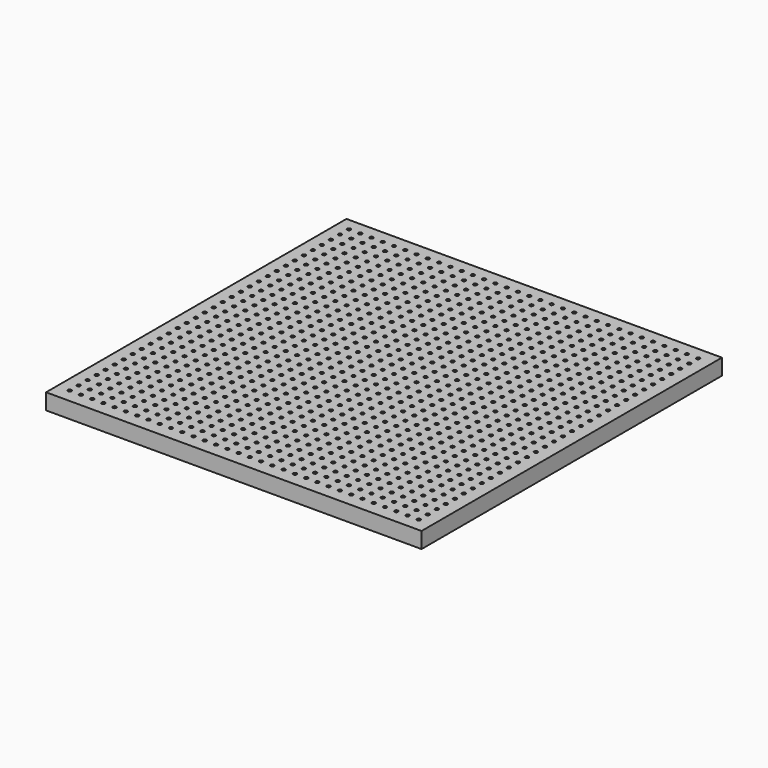
from build123d import *

# Parameters (mm, degrees)
F0_W     = 400
F0_H     = 400
F1_DEPTH = 1.5
F3_W     = 400
F3_H     = 400
F3_W_2   = 397
F3_H_2   = 397
F4_DEPTH = 15.5
F5_DEPTH = 10.5
F6_DEPTH = 10.5
F2_R     = 1.875
F7_DEPTH = 17.001


with BuildPart() as f1:
    # F0 (on Top) → F1 (new body)
    with BuildSketch(Plane.XY):
        Rectangle(F0_W, F0_H)
    extrude(amount=F1_DEPTH)

    # F3 (on face) → F4 (join)
    with BuildSketch(Plane(origin=(0, 0, 0), x_dir=(1, 0, 0), z_dir=(0, 0, -1))):
        Rectangle(F3_W, F3_H)
        Rectangle(F3_W_2, F3_H_2, mode=Mode.SUBTRACT)
    extrude(amount=F4_DEPTH)

    # F5 (add): a face of the model
    f5_faces = [f1.faces().sort_by_distance(p)[0] for p in [
        (0, -198.5, -7.75),
    ]]
    extrude(f5_faces, amount=F5_DEPTH)

    # F6 (add): a face of the model
    f6_faces = [f1.faces().sort_by_distance(p)[0] for p in [
        (0, 198.5, -7.75),
    ]]
    extrude(f6_faces, amount=F6_DEPTH)

    # F2 (on face) → F7 (cut, through all)
    with BuildSketch(Plane.XY.offset(1.5)):
        with Locations((-186.625, 186.625)):
            Circle(F2_R)
        with Locations((-186.625, 174.625)):
            Circle(F2_R)
        with Locations((-186.625, 162.625)):
            Circle(F2_R)
        with Locations((-186.625, 150.625)):
            Circle(F2_R)
        with Locations((-186.625, 138.625)):
            Circle(F2_R)
        with Locations((-186.625, 126.625)):
            Circle(F2_R)
        with Locations((-186.625, 114.625)):
            Circle(F2_R)
        with Locations((-186.625, 102.625)):
            Circle(F2_R)
        with Locations((-186.625, 90.625)):
            Circle(F2_R)
        with Locations((-186.625, 78.625)):
            Circle(F2_R)
        with Locations((-186.625, 66.625)):
            Circle(F2_R)
        with Locations((-186.625, 54.625)):
            Circle(F2_R)
        with Locations((-186.625, 42.625)):
            Circle(F2_R)
        with Locations((-186.625, 30.625)):
            Circle(F2_R)
        with Locations((-186.625, 18.625)):
            Circle(F2_R)
        with Locations((-186.625, 6.625)):
            Circle(F2_R)
        with Locations((-186.625, -5.375)):
            Circle(F2_R)
        with Locations((-186.625, -17.375)):
            Circle(F2_R)
        with Locations((-186.625, -29.375)):
            Circle(F2_R)
        with Locations((-186.625, -41.375)):
            Circle(F2_R)
        with Locations((-186.625, -53.375)):
            Circle(F2_R)
        with Locations((-186.625, -65.375)):
            Circle(F2_R)
        with Locations((-186.625, -77.375)):
            Circle(F2_R)
        with Locations((-186.625, -89.375)):
            Circle(F2_R)
        with Locations((-186.625, -101.375)):
            Circle(F2_R)
        with Locations((-186.625, -113.375)):
            Circle(F2_R)
        with Locations((-186.625, -125.375)):
            Circle(F2_R)
        with Locations((-186.625, -137.375)):
            Circle(F2_R)
        with Locations((-186.625, -149.375)):
            Circle(F2_R)
        with Locations((-186.625, -161.375)):
            Circle(F2_R)
        with Locations((-186.625, -173.375)):
            Circle(F2_R)
        with Locations((-186.625, -185.375)):
            Circle(F2_R)
        with Locations((-174.625, 186.625)):
            Circle(F2_R)
        with Locations((-174.625, 174.625)):
            Circle(F2_R)
        with Locations((-174.625, 162.625)):
            Circle(F2_R)
        with Locations((-174.625, 150.625)):
            Circle(F2_R)
        with Locations((-174.625, 138.625)):
            Circle(F2_R)
        with Locations((-174.625, 126.625)):
            Circle(F2_R)
        with Locations((-174.625, 114.625)):
            Circle(F2_R)
        with Locations((-174.625, 102.625)):
            Circle(F2_R)
        with Locations((-174.625, 90.625)):
            Circle(F2_R)
        with Locations((-174.625, 78.625)):
            Circle(F2_R)
        with Locations((-174.625, 66.625)):
            Circle(F2_R)
        with Locations((-174.625, 54.625)):
            Circle(F2_R)
        with Locations((-174.625, 42.625)):
            Circle(F2_R)
        with Locations((-174.625, 30.625)):
            Circle(F2_R)
        with Locations((-174.625, 18.625)):
            Circle(F2_R)
        with Locations((-174.625, 6.625)):
            Circle(F2_R)
        with Locations((-174.625, -5.375)):
            Circle(F2_R)
        with Locations((-174.625, -17.375)):
            Circle(F2_R)
        with Locations((-174.625, -29.375)):
            Circle(F2_R)
        with Locations((-174.625, -41.375)):
            Circle(F2_R)
        with Locations((-174.625, -53.375)):
            Circle(F2_R)
        with Locations((-174.625, -65.375)):
            Circle(F2_R)
        with Locations((-174.625, -77.375)):
            Circle(F2_R)
        with Locations((-174.625, -89.375)):
            Circle(F2_R)
        with Locations((-174.625, -101.375)):
            Circle(F2_R)
        with Locations((-174.625, -113.375)):
            Circle(F2_R)
        with Locations((-174.625, -125.375)):
            Circle(F2_R)
        with Locations((-174.625, -137.375)):
            Circle(F2_R)
        with Locations((-174.625, -149.375)):
            Circle(F2_R)
        with Locations((-174.625, -161.375)):
            Circle(F2_R)
        with Locations((-174.625, -173.375)):
            Circle(F2_R)
        with Locations((-174.625, -185.375)):
            Circle(F2_R)
        with Locations((-162.625, 186.625)):
            Circle(F2_R)
        with Locations((-162.625, 174.625)):
            Circle(F2_R)
        with Locations((-162.625, 162.625)):
            Circle(F2_R)
        with Locations((-162.625, 150.625)):
            Circle(F2_R)
        with Locations((-162.625, 138.625)):
            Circle(F2_R)
        with Locations((-162.625, 126.625)):
            Circle(F2_R)
        with Locations((-162.625, 114.625)):
            Circle(F2_R)
        with Locations((-162.625, 102.625)):
            Circle(F2_R)
        with Locations((-162.625, 90.625)):
            Circle(F2_R)
        with Locations((-162.625, 78.625)):
            Circle(F2_R)
        with Locations((-162.625, 66.625)):
            Circle(F2_R)
        with Locations((-162.625, 54.625)):
            Circle(F2_R)
        with Locations((-162.625, 42.625)):
            Circle(F2_R)
        with Locations((-162.625, 30.625)):
            Circle(F2_R)
        with Locations((-162.625, 18.625)):
            Circle(F2_R)
        with Locations((-162.625, 6.625)):
            Circle(F2_R)
        with Locations((-162.625, -5.375)):
            Circle(F2_R)
        with Locations((-162.625, -17.375)):
            Circle(F2_R)
        with Locations((-162.625, -29.375)):
            Circle(F2_R)
        with Locations((-162.625, -41.375)):
            Circle(F2_R)
        with Locations((-162.625, -53.375)):
            Circle(F2_R)
        with Locations((-162.625, -65.375)):
            Circle(F2_R)
        with Locations((-162.625, -77.375)):
            Circle(F2_R)
        with Locations((-162.625, -89.375)):
            Circle(F2_R)
        with Locations((-162.625, -101.375)):
            Circle(F2_R)
        with Locations((-162.625, -113.375)):
            Circle(F2_R)
        with Locations((-162.625, -125.375)):
            Circle(F2_R)
        with Locations((-162.625, -137.375)):
            Circle(F2_R)
        with Locations((-162.625, -149.375)):
            Circle(F2_R)
        with Locations((-162.625, -161.375)):
            Circle(F2_R)
        with Locations((-162.625, -173.375)):
            Circle(F2_R)
        with Locations((-162.625, -185.375)):
            Circle(F2_R)
        with Locations((-150.625, 186.625)):
            Circle(F2_R)
        with Locations((-150.625, 174.625)):
            Circle(F2_R)
        with Locations((-150.625, 162.625)):
            Circle(F2_R)
        with Locations((-150.625, 150.625)):
            Circle(F2_R)
        with Locations((-150.625, 138.625)):
            Circle(F2_R)
        with Locations((-150.625, 126.625)):
            Circle(F2_R)
        with Locations((-150.625, 114.625)):
            Circle(F2_R)
        with Locations((-150.625, 102.625)):
            Circle(F2_R)
        with Locations((-150.625, 90.625)):
            Circle(F2_R)
        with Locations((-150.625, 78.625)):
            Circle(F2_R)
        with Locations((-150.625, 66.625)):
            Circle(F2_R)
        with Locations((-150.625, 54.625)):
            Circle(F2_R)
        with Locations((-150.625, 42.625)):
            Circle(F2_R)
        with Locations((-150.625, 30.625)):
            Circle(F2_R)
        with Locations((-150.625, 18.625)):
            Circle(F2_R)
        with Locations((-150.625, 6.625)):
            Circle(F2_R)
        with Locations((-150.625, -5.375)):
            Circle(F2_R)
        with Locations((-150.625, -17.375)):
            Circle(F2_R)
        with Locations((-150.625, -29.375)):
            Circle(F2_R)
        with Locations((-150.625, -41.375)):
            Circle(F2_R)
        with Locations((-150.625, -53.375)):
            Circle(F2_R)
        with Locations((-150.625, -65.375)):
            Circle(F2_R)
        with Locations((-150.625, -77.375)):
            Circle(F2_R)
        with Locations((-150.625, -89.375)):
            Circle(F2_R)
        with Locations((-150.625, -101.375)):
            Circle(F2_R)
        with Locations((-150.625, -113.375)):
            Circle(F2_R)
        with Locations((-150.625, -125.375)):
            Circle(F2_R)
        with Locations((-150.625, -137.375)):
            Circle(F2_R)
        with Locations((-150.625, -149.375)):
            Circle(F2_R)
        with Locations((-150.625, -161.375)):
            Circle(F2_R)
        with Locations((-150.625, -173.375)):
            Circle(F2_R)
        with Locations((-150.625, -185.375)):
            Circle(F2_R)
        with Locations((-138.625, 186.625)):
            Circle(F2_R)
        with Locations((-138.625, 174.625)):
            Circle(F2_R)
        with Locations((-138.625, 162.625)):
            Circle(F2_R)
        with Locations((-138.625, 150.625)):
            Circle(F2_R)
        with Locations((-138.625, 138.625)):
            Circle(F2_R)
        with Locations((-138.625, 126.625)):
            Circle(F2_R)
        with Locations((-138.625, 114.625)):
            Circle(F2_R)
        with Locations((-138.625, 102.625)):
            Circle(F2_R)
        with Locations((-138.625, 90.625)):
            Circle(F2_R)
        with Locations((-138.625, 78.625)):
            Circle(F2_R)
        with Locations((-138.625, 66.625)):
            Circle(F2_R)
        with Locations((-138.625, 54.625)):
            Circle(F2_R)
        with Locations((-138.625, 42.625)):
            Circle(F2_R)
        with Locations((-138.625, 30.625)):
            Circle(F2_R)
        with Locations((-138.625, 18.625)):
            Circle(F2_R)
        with Locations((-138.625, 6.625)):
            Circle(F2_R)
        with Locations((-138.625, -5.375)):
            Circle(F2_R)
        with Locations((-138.625, -17.375)):
            Circle(F2_R)
        with Locations((-138.625, -29.375)):
            Circle(F2_R)
        with Locations((-138.625, -41.375)):
            Circle(F2_R)
        with Locations((-138.625, -53.375)):
            Circle(F2_R)
        with Locations((-138.625, -65.375)):
            Circle(F2_R)
        with Locations((-138.625, -77.375)):
            Circle(F2_R)
        with Locations((-138.625, -89.375)):
            Circle(F2_R)
        with Locations((-138.625, -101.375)):
            Circle(F2_R)
        with Locations((-138.625, -113.375)):
            Circle(F2_R)
        with Locations((-138.625, -125.375)):
            Circle(F2_R)
        with Locations((-138.625, -137.375)):
            Circle(F2_R)
        with Locations((-138.625, -149.375)):
            Circle(F2_R)
        with Locations((-138.625, -161.375)):
            Circle(F2_R)
        with Locations((-138.625, -173.375)):
            Circle(F2_R)
        with Locations((-138.625, -185.375)):
            Circle(F2_R)
        with Locations((-126.625, 186.625)):
            Circle(F2_R)
        with Locations((-126.625, 174.625)):
            Circle(F2_R)
        with Locations((-126.625, 162.625)):
            Circle(F2_R)
        with Locations((-126.625, 150.625)):
            Circle(F2_R)
        with Locations((-126.625, 138.625)):
            Circle(F2_R)
        with Locations((-126.625, 126.625)):
            Circle(F2_R)
        with Locations((-126.625, 114.625)):
            Circle(F2_R)
        with Locations((-126.625, 102.625)):
            Circle(F2_R)
        with Locations((-126.625, 90.625)):
            Circle(F2_R)
        with Locations((-126.625, 78.625)):
            Circle(F2_R)
        with Locations((-126.625, 66.625)):
            Circle(F2_R)
        with Locations((-126.625, 54.625)):
            Circle(F2_R)
        with Locations((-126.625, 42.625)):
            Circle(F2_R)
        with Locations((-126.625, 30.625)):
            Circle(F2_R)
        with Locations((-126.625, 18.625)):
            Circle(F2_R)
        with Locations((-126.625, 6.625)):
            Circle(F2_R)
        with Locations((-126.625, -5.375)):
            Circle(F2_R)
        with Locations((-126.625, -17.375)):
            Circle(F2_R)
        with Locations((-126.625, -29.375)):
            Circle(F2_R)
        with Locations((-126.625, -41.375)):
            Circle(F2_R)
        with Locations((-126.625, -53.375)):
            Circle(F2_R)
        with Locations((-126.625, -65.375)):
            Circle(F2_R)
        with Locations((-126.625, -77.375)):
            Circle(F2_R)
        with Locations((-126.625, -89.375)):
            Circle(F2_R)
        with Locations((-126.625, -101.375)):
            Circle(F2_R)
        with Locations((-126.625, -113.375)):
            Circle(F2_R)
        with Locations((-126.625, -125.375)):
            Circle(F2_R)
        with Locations((-126.625, -137.375)):
            Circle(F2_R)
        with Locations((-126.625, -149.375)):
            Circle(F2_R)
        with Locations((-126.625, -161.375)):
            Circle(F2_R)
        with Locations((-126.625, -173.375)):
            Circle(F2_R)
        with Locations((-126.625, -185.375)):
            Circle(F2_R)
        with Locations((-114.625, 186.625)):
            Circle(F2_R)
        with Locations((-114.625, 174.625)):
            Circle(F2_R)
        with Locations((-114.625, 162.625)):
            Circle(F2_R)
        with Locations((-114.625, 150.625)):
            Circle(F2_R)
        with Locations((-114.625, 138.625)):
            Circle(F2_R)
        with Locations((-114.625, 126.625)):
            Circle(F2_R)
        with Locations((-114.625, 114.625)):
            Circle(F2_R)
        with Locations((-114.625, 102.625)):
            Circle(F2_R)
        with Locations((-114.625, 90.625)):
            Circle(F2_R)
        with Locations((-114.625, 78.625)):
            Circle(F2_R)
        with Locations((-114.625, 66.625)):
            Circle(F2_R)
        with Locations((-114.625, 54.625)):
            Circle(F2_R)
        with Locations((-114.625, 42.625)):
            Circle(F2_R)
        with Locations((-114.625, 30.625)):
            Circle(F2_R)
        with Locations((-114.625, 18.625)):
            Circle(F2_R)
        with Locations((-114.625, 6.625)):
            Circle(F2_R)
        with Locations((-114.625, -5.375)):
            Circle(F2_R)
        with Locations((-114.625, -17.375)):
            Circle(F2_R)
        with Locations((-114.625, -29.375)):
            Circle(F2_R)
        with Locations((-114.625, -41.375)):
            Circle(F2_R)
        with Locations((-114.625, -53.375)):
            Circle(F2_R)
        with Locations((-114.625, -65.375)):
            Circle(F2_R)
        with Locations((-114.625, -77.375)):
            Circle(F2_R)
        with Locations((-114.625, -89.375)):
            Circle(F2_R)
        with Locations((-114.625, -101.375)):
            Circle(F2_R)
        with Locations((-114.625, -113.375)):
            Circle(F2_R)
        with Locations((-114.625, -125.375)):
            Circle(F2_R)
        with Locations((-114.625, -137.375)):
            Circle(F2_R)
        with Locations((-114.625, -149.375)):
            Circle(F2_R)
        with Locations((-114.625, -161.375)):
            Circle(F2_R)
        with Locations((-114.625, -173.375)):
            Circle(F2_R)
        with Locations((-114.625, -185.375)):
            Circle(F2_R)
        with Locations((-102.625, 186.625)):
            Circle(F2_R)
        with Locations((-102.625, 174.625)):
            Circle(F2_R)
        with Locations((-102.625, 162.625)):
            Circle(F2_R)
        with Locations((-102.625, 150.625)):
            Circle(F2_R)
        with Locations((-102.625, 138.625)):
            Circle(F2_R)
        with Locations((-102.625, 126.625)):
            Circle(F2_R)
        with Locations((-102.625, 114.625)):
            Circle(F2_R)
        with Locations((-102.625, 102.625)):
            Circle(F2_R)
        with Locations((-102.625, 90.625)):
            Circle(F2_R)
        with Locations((-102.625, 78.625)):
            Circle(F2_R)
        with Locations((-102.625, 66.625)):
            Circle(F2_R)
        with Locations((-102.625, 54.625)):
            Circle(F2_R)
        with Locations((-102.625, 42.625)):
            Circle(F2_R)
        with Locations((-102.625, 30.625)):
            Circle(F2_R)
        with Locations((-102.625, 18.625)):
            Circle(F2_R)
        with Locations((-102.625, 6.625)):
            Circle(F2_R)
        with Locations((-102.625, -5.375)):
            Circle(F2_R)
        with Locations((-102.625, -17.375)):
            Circle(F2_R)
        with Locations((-102.625, -29.375)):
            Circle(F2_R)
        with Locations((-102.625, -41.375)):
            Circle(F2_R)
        with Locations((-102.625, -53.375)):
            Circle(F2_R)
        with Locations((-102.625, -65.375)):
            Circle(F2_R)
        with Locations((-102.625, -77.375)):
            Circle(F2_R)
        with Locations((-102.625, -89.375)):
            Circle(F2_R)
        with Locations((-102.625, -101.375)):
            Circle(F2_R)
        with Locations((-102.625, -113.375)):
            Circle(F2_R)
        with Locations((-102.625, -125.375)):
            Circle(F2_R)
        with Locations((-102.625, -137.375)):
            Circle(F2_R)
        with Locations((-102.625, -149.375)):
            Circle(F2_R)
        with Locations((-102.625, -161.375)):
            Circle(F2_R)
        with Locations((-102.625, -173.375)):
            Circle(F2_R)
        with Locations((-102.625, -185.375)):
            Circle(F2_R)
        with Locations((-90.625, 186.625)):
            Circle(F2_R)
        with Locations((-90.625, 174.625)):
            Circle(F2_R)
        with Locations((-90.625, 162.625)):
            Circle(F2_R)
        with Locations((-90.625, 150.625)):
            Circle(F2_R)
        with Locations((-90.625, 138.625)):
            Circle(F2_R)
        with Locations((-90.625, 126.625)):
            Circle(F2_R)
        with Locations((-90.625, 114.625)):
            Circle(F2_R)
        with Locations((-90.625, 102.625)):
            Circle(F2_R)
        with Locations((-90.625, 90.625)):
            Circle(F2_R)
        with Locations((-90.625, 78.625)):
            Circle(F2_R)
        with Locations((-90.625, 66.625)):
            Circle(F2_R)
        with Locations((-90.625, 54.625)):
            Circle(F2_R)
        with Locations((-90.625, 42.625)):
            Circle(F2_R)
        with Locations((-90.625, 30.625)):
            Circle(F2_R)
        with Locations((-90.625, 18.625)):
            Circle(F2_R)
        with Locations((-90.625, 6.625)):
            Circle(F2_R)
        with Locations((-90.625, -5.375)):
            Circle(F2_R)
        with Locations((-90.625, -17.375)):
            Circle(F2_R)
        with Locations((-90.625, -29.375)):
            Circle(F2_R)
        with Locations((-90.625, -41.375)):
            Circle(F2_R)
        with Locations((-90.625, -53.375)):
            Circle(F2_R)
        with Locations((-90.625, -65.375)):
            Circle(F2_R)
        with Locations((-90.625, -77.375)):
            Circle(F2_R)
        with Locations((-90.625, -89.375)):
            Circle(F2_R)
        with Locations((-90.625, -101.375)):
            Circle(F2_R)
        with Locations((-90.625, -113.375)):
            Circle(F2_R)
        with Locations((-90.625, -125.375)):
            Circle(F2_R)
        with Locations((-90.625, -137.375)):
            Circle(F2_R)
        with Locations((-90.625, -149.375)):
            Circle(F2_R)
        with Locations((-90.625, -161.375)):
            Circle(F2_R)
        with Locations((-90.625, -173.375)):
            Circle(F2_R)
        with Locations((-90.625, -185.375)):
            Circle(F2_R)
        with Locations((-78.625, 186.625)):
            Circle(F2_R)
        with Locations((-78.625, 174.625)):
            Circle(F2_R)
        with Locations((-78.625, 162.625)):
            Circle(F2_R)
        with Locations((-78.625, 150.625)):
            Circle(F2_R)
        with Locations((-78.625, 138.625)):
            Circle(F2_R)
        with Locations((-78.625, 126.625)):
            Circle(F2_R)
        with Locations((-78.625, 114.625)):
            Circle(F2_R)
        with Locations((-78.625, 102.625)):
            Circle(F2_R)
        with Locations((-78.625, 90.625)):
            Circle(F2_R)
        with Locations((-78.625, 78.625)):
            Circle(F2_R)
        with Locations((-78.625, 66.625)):
            Circle(F2_R)
        with Locations((-78.625, 54.625)):
            Circle(F2_R)
        with Locations((-78.625, 42.625)):
            Circle(F2_R)
        with Locations((-78.625, 30.625)):
            Circle(F2_R)
        with Locations((-78.625, 18.625)):
            Circle(F2_R)
        with Locations((-78.625, 6.625)):
            Circle(F2_R)
        with Locations((-78.625, -5.375)):
            Circle(F2_R)
        with Locations((-78.625, -17.375)):
            Circle(F2_R)
        with Locations((-78.625, -29.375)):
            Circle(F2_R)
        with Locations((-78.625, -41.375)):
            Circle(F2_R)
        with Locations((-78.625, -53.375)):
            Circle(F2_R)
        with Locations((-78.625, -65.375)):
            Circle(F2_R)
        with Locations((-78.625, -77.375)):
            Circle(F2_R)
        with Locations((-78.625, -89.375)):
            Circle(F2_R)
        with Locations((-78.625, -101.375)):
            Circle(F2_R)
        with Locations((-78.625, -113.375)):
            Circle(F2_R)
        with Locations((-78.625, -125.375)):
            Circle(F2_R)
        with Locations((-78.625, -137.375)):
            Circle(F2_R)
        with Locations((-78.625, -149.375)):
            Circle(F2_R)
        with Locations((-78.625, -161.375)):
            Circle(F2_R)
        with Locations((-78.625, -173.375)):
            Circle(F2_R)
        with Locations((-78.625, -185.375)):
            Circle(F2_R)
        with Locations((-66.625, 186.625)):
            Circle(F2_R)
        with Locations((-66.625, 174.625)):
            Circle(F2_R)
        with Locations((-66.625, 162.625)):
            Circle(F2_R)
        with Locations((-66.625, 150.625)):
            Circle(F2_R)
        with Locations((-66.625, 138.625)):
            Circle(F2_R)
        with Locations((-66.625, 126.625)):
            Circle(F2_R)
        with Locations((-66.625, 114.625)):
            Circle(F2_R)
        with Locations((-66.625, 102.625)):
            Circle(F2_R)
        with Locations((-66.625, 90.625)):
            Circle(F2_R)
        with Locations((-66.625, 78.625)):
            Circle(F2_R)
        with Locations((-66.625, 66.625)):
            Circle(F2_R)
        with Locations((-66.625, 54.625)):
            Circle(F2_R)
        with Locations((-66.625, 42.625)):
            Circle(F2_R)
        with Locations((-66.625, 30.625)):
            Circle(F2_R)
        with Locations((-66.625, 18.625)):
            Circle(F2_R)
        with Locations((-66.625, 6.625)):
            Circle(F2_R)
        with Locations((-66.625, -5.375)):
            Circle(F2_R)
        with Locations((-66.625, -17.375)):
            Circle(F2_R)
        with Locations((-66.625, -29.375)):
            Circle(F2_R)
        with Locations((-66.625, -41.375)):
            Circle(F2_R)
        with Locations((-66.625, -53.375)):
            Circle(F2_R)
        with Locations((-66.625, -65.375)):
            Circle(F2_R)
        with Locations((-66.625, -77.375)):
            Circle(F2_R)
        with Locations((-66.625, -89.375)):
            Circle(F2_R)
        with Locations((-66.625, -101.375)):
            Circle(F2_R)
        with Locations((-66.625, -113.375)):
            Circle(F2_R)
        with Locations((-66.625, -125.375)):
            Circle(F2_R)
        with Locations((-66.625, -137.375)):
            Circle(F2_R)
        with Locations((-66.625, -149.375)):
            Circle(F2_R)
        with Locations((-66.625, -161.375)):
            Circle(F2_R)
        with Locations((-66.625, -173.375)):
            Circle(F2_R)
        with Locations((-66.625, -185.375)):
            Circle(F2_R)
        with Locations((-54.625, 186.625)):
            Circle(F2_R)
        with Locations((-54.625, 174.625)):
            Circle(F2_R)
        with Locations((-54.625, 162.625)):
            Circle(F2_R)
        with Locations((-54.625, 150.625)):
            Circle(F2_R)
        with Locations((-54.625, 138.625)):
            Circle(F2_R)
        with Locations((-54.625, 126.625)):
            Circle(F2_R)
        with Locations((-54.625, 114.625)):
            Circle(F2_R)
        with Locations((-54.625, 102.625)):
            Circle(F2_R)
        with Locations((-54.625, 90.625)):
            Circle(F2_R)
        with Locations((-54.625, 78.625)):
            Circle(F2_R)
        with Locations((-54.625, 66.625)):
            Circle(F2_R)
        with Locations((-54.625, 54.625)):
            Circle(F2_R)
        with Locations((-54.625, 42.625)):
            Circle(F2_R)
        with Locations((-54.625, 30.625)):
            Circle(F2_R)
        with Locations((-54.625, 18.625)):
            Circle(F2_R)
        with Locations((-54.625, 6.625)):
            Circle(F2_R)
        with Locations((-54.625, -5.375)):
            Circle(F2_R)
        with Locations((-54.625, -17.375)):
            Circle(F2_R)
        with Locations((-54.625, -29.375)):
            Circle(F2_R)
        with Locations((-54.625, -41.375)):
            Circle(F2_R)
        with Locations((-54.625, -53.375)):
            Circle(F2_R)
        with Locations((-54.625, -65.375)):
            Circle(F2_R)
        with Locations((-54.625, -77.375)):
            Circle(F2_R)
        with Locations((-54.625, -89.375)):
            Circle(F2_R)
        with Locations((-54.625, -101.375)):
            Circle(F2_R)
        with Locations((-54.625, -113.375)):
            Circle(F2_R)
        with Locations((-54.625, -125.375)):
            Circle(F2_R)
        with Locations((-54.625, -137.375)):
            Circle(F2_R)
        with Locations((-54.625, -149.375)):
            Circle(F2_R)
        with Locations((-54.625, -161.375)):
            Circle(F2_R)
        with Locations((-54.625, -173.375)):
            Circle(F2_R)
        with Locations((-54.625, -185.375)):
            Circle(F2_R)
        with Locations((-42.625, 186.625)):
            Circle(F2_R)
        with Locations((-42.625, 174.625)):
            Circle(F2_R)
        with Locations((-42.625, 162.625)):
            Circle(F2_R)
        with Locations((-42.625, 150.625)):
            Circle(F2_R)
        with Locations((-42.625, 138.625)):
            Circle(F2_R)
        with Locations((-42.625, 126.625)):
            Circle(F2_R)
        with Locations((-42.625, 114.625)):
            Circle(F2_R)
        with Locations((-42.625, 102.625)):
            Circle(F2_R)
        with Locations((-42.625, 90.625)):
            Circle(F2_R)
        with Locations((-42.625, 78.625)):
            Circle(F2_R)
        with Locations((-42.625, 66.625)):
            Circle(F2_R)
        with Locations((-42.625, 54.625)):
            Circle(F2_R)
        with Locations((-42.625, 42.625)):
            Circle(F2_R)
        with Locations((-42.625, 30.625)):
            Circle(F2_R)
        with Locations((-42.625, 18.625)):
            Circle(F2_R)
        with Locations((-42.625, 6.625)):
            Circle(F2_R)
        with Locations((-42.625, -5.375)):
            Circle(F2_R)
        with Locations((-42.625, -17.375)):
            Circle(F2_R)
        with Locations((-42.625, -29.375)):
            Circle(F2_R)
        with Locations((-42.625, -41.375)):
            Circle(F2_R)
        with Locations((-42.625, -53.375)):
            Circle(F2_R)
        with Locations((-42.625, -65.375)):
            Circle(F2_R)
        with Locations((-42.625, -77.375)):
            Circle(F2_R)
        with Locations((-42.625, -89.375)):
            Circle(F2_R)
        with Locations((-42.625, -101.375)):
            Circle(F2_R)
        with Locations((-42.625, -113.375)):
            Circle(F2_R)
        with Locations((-42.625, -125.375)):
            Circle(F2_R)
        with Locations((-42.625, -137.375)):
            Circle(F2_R)
        with Locations((-42.625, -149.375)):
            Circle(F2_R)
        with Locations((-42.625, -161.375)):
            Circle(F2_R)
        with Locations((-42.625, -173.375)):
            Circle(F2_R)
        with Locations((-42.625, -185.375)):
            Circle(F2_R)
        with Locations((-30.625, 186.625)):
            Circle(F2_R)
        with Locations((-30.625, 174.625)):
            Circle(F2_R)
        with Locations((-30.625, 162.625)):
            Circle(F2_R)
        with Locations((-30.625, 150.625)):
            Circle(F2_R)
        with Locations((-30.625, 138.625)):
            Circle(F2_R)
        with Locations((-30.625, 126.625)):
            Circle(F2_R)
        with Locations((-30.625, 114.625)):
            Circle(F2_R)
        with Locations((-30.625, 102.625)):
            Circle(F2_R)
        with Locations((-30.625, 90.625)):
            Circle(F2_R)
        with Locations((-30.625, 78.625)):
            Circle(F2_R)
        with Locations((-30.625, 66.625)):
            Circle(F2_R)
        with Locations((-30.625, 54.625)):
            Circle(F2_R)
        with Locations((-30.625, 42.625)):
            Circle(F2_R)
        with Locations((-30.625, 30.625)):
            Circle(F2_R)
        with Locations((-30.625, 18.625)):
            Circle(F2_R)
        with Locations((-30.625, 6.625)):
            Circle(F2_R)
        with Locations((-30.625, -5.375)):
            Circle(F2_R)
        with Locations((-30.625, -17.375)):
            Circle(F2_R)
        with Locations((-30.625, -29.375)):
            Circle(F2_R)
        with Locations((-30.625, -41.375)):
            Circle(F2_R)
        with Locations((-30.625, -53.375)):
            Circle(F2_R)
        with Locations((-30.625, -65.375)):
            Circle(F2_R)
        with Locations((-30.625, -77.375)):
            Circle(F2_R)
        with Locations((-30.625, -89.375)):
            Circle(F2_R)
        with Locations((-30.625, -101.375)):
            Circle(F2_R)
        with Locations((-30.625, -113.375)):
            Circle(F2_R)
        with Locations((-30.625, -125.375)):
            Circle(F2_R)
        with Locations((-30.625, -137.375)):
            Circle(F2_R)
        with Locations((-30.625, -149.375)):
            Circle(F2_R)
        with Locations((-30.625, -161.375)):
            Circle(F2_R)
        with Locations((-30.625, -173.375)):
            Circle(F2_R)
        with Locations((-30.625, -185.375)):
            Circle(F2_R)
        with Locations((-18.625, 186.625)):
            Circle(F2_R)
        with Locations((-18.625, 174.625)):
            Circle(F2_R)
        with Locations((-18.625, 162.625)):
            Circle(F2_R)
        with Locations((-18.625, 150.625)):
            Circle(F2_R)
        with Locations((-18.625, 138.625)):
            Circle(F2_R)
        with Locations((-18.625, 126.625)):
            Circle(F2_R)
        with Locations((-18.625, 114.625)):
            Circle(F2_R)
        with Locations((-18.625, 102.625)):
            Circle(F2_R)
        with Locations((-18.625, 90.625)):
            Circle(F2_R)
        with Locations((-18.625, 78.625)):
            Circle(F2_R)
        with Locations((-18.625, 66.625)):
            Circle(F2_R)
        with Locations((-18.625, 54.625)):
            Circle(F2_R)
        with Locations((-18.625, 42.625)):
            Circle(F2_R)
        with Locations((-18.625, 30.625)):
            Circle(F2_R)
        with Locations((-18.625, 18.625)):
            Circle(F2_R)
        with Locations((-18.625, 6.625)):
            Circle(F2_R)
        with Locations((-18.625, -5.375)):
            Circle(F2_R)
        with Locations((-18.625, -17.375)):
            Circle(F2_R)
        with Locations((-18.625, -29.375)):
            Circle(F2_R)
        with Locations((-18.625, -41.375)):
            Circle(F2_R)
        with Locations((-18.625, -53.375)):
            Circle(F2_R)
        with Locations((-18.625, -65.375)):
            Circle(F2_R)
        with Locations((-18.625, -77.375)):
            Circle(F2_R)
        with Locations((-18.625, -89.375)):
            Circle(F2_R)
        with Locations((-18.625, -101.375)):
            Circle(F2_R)
        with Locations((-18.625, -113.375)):
            Circle(F2_R)
        with Locations((-18.625, -125.375)):
            Circle(F2_R)
        with Locations((-18.625, -137.375)):
            Circle(F2_R)
        with Locations((-18.625, -149.375)):
            Circle(F2_R)
        with Locations((-18.625, -161.375)):
            Circle(F2_R)
        with Locations((-18.625, -173.375)):
            Circle(F2_R)
        with Locations((-18.625, -185.375)):
            Circle(F2_R)
        with Locations((-6.625, 186.625)):
            Circle(F2_R)
        with Locations((-6.625, 174.625)):
            Circle(F2_R)
        with Locations((-6.625, 162.625)):
            Circle(F2_R)
        with Locations((-6.625, 150.625)):
            Circle(F2_R)
        with Locations((-6.625, 138.625)):
            Circle(F2_R)
        with Locations((-6.625, 126.625)):
            Circle(F2_R)
        with Locations((-6.625, 114.625)):
            Circle(F2_R)
        with Locations((-6.625, 102.625)):
            Circle(F2_R)
        with Locations((-6.625, 90.625)):
            Circle(F2_R)
        with Locations((-6.625, 78.625)):
            Circle(F2_R)
        with Locations((-6.625, 66.625)):
            Circle(F2_R)
        with Locations((-6.625, 54.625)):
            Circle(F2_R)
        with Locations((-6.625, 42.625)):
            Circle(F2_R)
        with Locations((-6.625, 30.625)):
            Circle(F2_R)
        with Locations((-6.625, 18.625)):
            Circle(F2_R)
        with Locations((-6.625, 6.625)):
            Circle(F2_R)
        with Locations((-6.625, -5.375)):
            Circle(F2_R)
        with Locations((-6.625, -17.375)):
            Circle(F2_R)
        with Locations((-6.625, -29.375)):
            Circle(F2_R)
        with Locations((-6.625, -41.375)):
            Circle(F2_R)
        with Locations((-6.625, -53.375)):
            Circle(F2_R)
        with Locations((-6.625, -65.375)):
            Circle(F2_R)
        with Locations((-6.625, -77.375)):
            Circle(F2_R)
        with Locations((-6.625, -89.375)):
            Circle(F2_R)
        with Locations((-6.625, -101.375)):
            Circle(F2_R)
        with Locations((-6.625, -113.375)):
            Circle(F2_R)
        with Locations((-6.625, -125.375)):
            Circle(F2_R)
        with Locations((-6.625, -137.375)):
            Circle(F2_R)
        with Locations((-6.625, -149.375)):
            Circle(F2_R)
        with Locations((-6.625, -161.375)):
            Circle(F2_R)
        with Locations((-6.625, -173.375)):
            Circle(F2_R)
        with Locations((-6.625, -185.375)):
            Circle(F2_R)
        with Locations((5.375, 186.625)):
            Circle(F2_R)
        with Locations((5.375, 174.625)):
            Circle(F2_R)
        with Locations((5.375, 162.625)):
            Circle(F2_R)
        with Locations((5.375, 150.625)):
            Circle(F2_R)
        with Locations((5.375, 138.625)):
            Circle(F2_R)
        with Locations((5.375, 126.625)):
            Circle(F2_R)
        with Locations((5.375, 114.625)):
            Circle(F2_R)
        with Locations((5.375, 102.625)):
            Circle(F2_R)
        with Locations((5.375, 90.625)):
            Circle(F2_R)
        with Locations((5.375, 78.625)):
            Circle(F2_R)
        with Locations((5.375, 66.625)):
            Circle(F2_R)
        with Locations((5.375, 54.625)):
            Circle(F2_R)
        with Locations((5.375, 42.625)):
            Circle(F2_R)
        with Locations((5.375, 30.625)):
            Circle(F2_R)
        with Locations((5.375, 18.625)):
            Circle(F2_R)
        with Locations((5.375, 6.625)):
            Circle(F2_R)
        with Locations((5.375, -5.375)):
            Circle(F2_R)
        with Locations((5.375, -17.375)):
            Circle(F2_R)
        with Locations((5.375, -29.375)):
            Circle(F2_R)
        with Locations((5.375, -41.375)):
            Circle(F2_R)
        with Locations((5.375, -53.375)):
            Circle(F2_R)
        with Locations((5.375, -65.375)):
            Circle(F2_R)
        with Locations((5.375, -77.375)):
            Circle(F2_R)
        with Locations((5.375, -89.375)):
            Circle(F2_R)
        with Locations((5.375, -101.375)):
            Circle(F2_R)
        with Locations((5.375, -113.375)):
            Circle(F2_R)
        with Locations((5.375, -125.375)):
            Circle(F2_R)
        with Locations((5.375, -137.375)):
            Circle(F2_R)
        with Locations((5.375, -149.375)):
            Circle(F2_R)
        with Locations((5.375, -161.375)):
            Circle(F2_R)
        with Locations((5.375, -173.375)):
            Circle(F2_R)
        with Locations((5.375, -185.375)):
            Circle(F2_R)
        with Locations((17.375, 186.625)):
            Circle(F2_R)
        with Locations((17.375, 174.625)):
            Circle(F2_R)
        with Locations((17.375, 162.625)):
            Circle(F2_R)
        with Locations((17.375, 150.625)):
            Circle(F2_R)
        with Locations((17.375, 138.625)):
            Circle(F2_R)
        with Locations((17.375, 126.625)):
            Circle(F2_R)
        with Locations((17.375, 114.625)):
            Circle(F2_R)
        with Locations((17.375, 102.625)):
            Circle(F2_R)
        with Locations((17.375, 90.625)):
            Circle(F2_R)
        with Locations((17.375, 78.625)):
            Circle(F2_R)
        with Locations((17.375, 66.625)):
            Circle(F2_R)
        with Locations((17.375, 54.625)):
            Circle(F2_R)
        with Locations((17.375, 42.625)):
            Circle(F2_R)
        with Locations((17.375, 30.625)):
            Circle(F2_R)
        with Locations((17.375, 18.625)):
            Circle(F2_R)
        with Locations((17.375, 6.625)):
            Circle(F2_R)
        with Locations((17.375, -5.375)):
            Circle(F2_R)
        with Locations((17.375, -17.375)):
            Circle(F2_R)
        with Locations((17.375, -29.375)):
            Circle(F2_R)
        with Locations((17.375, -41.375)):
            Circle(F2_R)
        with Locations((17.375, -53.375)):
            Circle(F2_R)
        with Locations((17.375, -65.375)):
            Circle(F2_R)
        with Locations((17.375, -77.375)):
            Circle(F2_R)
        with Locations((17.375, -89.375)):
            Circle(F2_R)
        with Locations((17.375, -101.375)):
            Circle(F2_R)
        with Locations((17.375, -113.375)):
            Circle(F2_R)
        with Locations((17.375, -125.375)):
            Circle(F2_R)
        with Locations((17.375, -137.375)):
            Circle(F2_R)
        with Locations((17.375, -149.375)):
            Circle(F2_R)
        with Locations((17.375, -161.375)):
            Circle(F2_R)
        with Locations((17.375, -173.375)):
            Circle(F2_R)
        with Locations((17.375, -185.375)):
            Circle(F2_R)
        with Locations((29.375, 186.625)):
            Circle(F2_R)
        with Locations((29.375, 174.625)):
            Circle(F2_R)
        with Locations((29.375, 162.625)):
            Circle(F2_R)
        with Locations((29.375, 150.625)):
            Circle(F2_R)
        with Locations((29.375, 138.625)):
            Circle(F2_R)
        with Locations((29.375, 126.625)):
            Circle(F2_R)
        with Locations((29.375, 114.625)):
            Circle(F2_R)
        with Locations((29.375, 102.625)):
            Circle(F2_R)
        with Locations((29.375, 90.625)):
            Circle(F2_R)
        with Locations((29.375, 78.625)):
            Circle(F2_R)
        with Locations((29.375, 66.625)):
            Circle(F2_R)
        with Locations((29.375, 54.625)):
            Circle(F2_R)
        with Locations((29.375, 42.625)):
            Circle(F2_R)
        with Locations((29.375, 30.625)):
            Circle(F2_R)
        with Locations((29.375, 18.625)):
            Circle(F2_R)
        with Locations((29.375, 6.625)):
            Circle(F2_R)
        with Locations((29.375, -5.375)):
            Circle(F2_R)
        with Locations((29.375, -17.375)):
            Circle(F2_R)
        with Locations((29.375, -29.375)):
            Circle(F2_R)
        with Locations((29.375, -41.375)):
            Circle(F2_R)
        with Locations((29.375, -53.375)):
            Circle(F2_R)
        with Locations((29.375, -65.375)):
            Circle(F2_R)
        with Locations((29.375, -77.375)):
            Circle(F2_R)
        with Locations((29.375, -89.375)):
            Circle(F2_R)
        with Locations((29.375, -101.375)):
            Circle(F2_R)
        with Locations((29.375, -113.375)):
            Circle(F2_R)
        with Locations((29.375, -125.375)):
            Circle(F2_R)
        with Locations((29.375, -137.375)):
            Circle(F2_R)
        with Locations((29.375, -149.375)):
            Circle(F2_R)
        with Locations((29.375, -161.375)):
            Circle(F2_R)
        with Locations((29.375, -173.375)):
            Circle(F2_R)
        with Locations((29.375, -185.375)):
            Circle(F2_R)
        with Locations((41.375, 186.625)):
            Circle(F2_R)
        with Locations((41.375, 174.625)):
            Circle(F2_R)
        with Locations((41.375, 162.625)):
            Circle(F2_R)
        with Locations((41.375, 150.625)):
            Circle(F2_R)
        with Locations((41.375, 138.625)):
            Circle(F2_R)
        with Locations((41.375, 126.625)):
            Circle(F2_R)
        with Locations((41.375, 114.625)):
            Circle(F2_R)
        with Locations((41.375, 102.625)):
            Circle(F2_R)
        with Locations((41.375, 90.625)):
            Circle(F2_R)
        with Locations((41.375, 78.625)):
            Circle(F2_R)
        with Locations((41.375, 66.625)):
            Circle(F2_R)
        with Locations((41.375, 54.625)):
            Circle(F2_R)
        with Locations((41.375, 42.625)):
            Circle(F2_R)
        with Locations((41.375, 30.625)):
            Circle(F2_R)
        with Locations((41.375, 18.625)):
            Circle(F2_R)
        with Locations((41.375, 6.625)):
            Circle(F2_R)
        with Locations((41.375, -5.375)):
            Circle(F2_R)
        with Locations((41.375, -17.375)):
            Circle(F2_R)
        with Locations((41.375, -29.375)):
            Circle(F2_R)
        with Locations((41.375, -41.375)):
            Circle(F2_R)
        with Locations((41.375, -53.375)):
            Circle(F2_R)
        with Locations((41.375, -65.375)):
            Circle(F2_R)
        with Locations((41.375, -77.375)):
            Circle(F2_R)
        with Locations((41.375, -89.375)):
            Circle(F2_R)
        with Locations((41.375, -101.375)):
            Circle(F2_R)
        with Locations((41.375, -113.375)):
            Circle(F2_R)
        with Locations((41.375, -125.375)):
            Circle(F2_R)
        with Locations((41.375, -137.375)):
            Circle(F2_R)
        with Locations((41.375, -149.375)):
            Circle(F2_R)
        with Locations((41.375, -161.375)):
            Circle(F2_R)
        with Locations((41.375, -173.375)):
            Circle(F2_R)
        with Locations((41.375, -185.375)):
            Circle(F2_R)
        with Locations((53.375, 186.625)):
            Circle(F2_R)
        with Locations((53.375, 174.625)):
            Circle(F2_R)
        with Locations((53.375, 162.625)):
            Circle(F2_R)
        with Locations((53.375, 150.625)):
            Circle(F2_R)
        with Locations((53.375, 138.625)):
            Circle(F2_R)
        with Locations((53.375, 126.625)):
            Circle(F2_R)
        with Locations((53.375, 114.625)):
            Circle(F2_R)
        with Locations((53.375, 102.625)):
            Circle(F2_R)
        with Locations((53.375, 90.625)):
            Circle(F2_R)
        with Locations((53.375, 78.625)):
            Circle(F2_R)
        with Locations((53.375, 66.625)):
            Circle(F2_R)
        with Locations((53.375, 54.625)):
            Circle(F2_R)
        with Locations((53.375, 42.625)):
            Circle(F2_R)
        with Locations((53.375, 30.625)):
            Circle(F2_R)
        with Locations((53.375, 18.625)):
            Circle(F2_R)
        with Locations((53.375, 6.625)):
            Circle(F2_R)
        with Locations((53.375, -5.375)):
            Circle(F2_R)
        with Locations((53.375, -17.375)):
            Circle(F2_R)
        with Locations((53.375, -29.375)):
            Circle(F2_R)
        with Locations((53.375, -41.375)):
            Circle(F2_R)
        with Locations((53.375, -53.375)):
            Circle(F2_R)
        with Locations((53.375, -65.375)):
            Circle(F2_R)
        with Locations((53.375, -77.375)):
            Circle(F2_R)
        with Locations((53.375, -89.375)):
            Circle(F2_R)
        with Locations((53.375, -101.375)):
            Circle(F2_R)
        with Locations((53.375, -113.375)):
            Circle(F2_R)
        with Locations((53.375, -125.375)):
            Circle(F2_R)
        with Locations((53.375, -137.375)):
            Circle(F2_R)
        with Locations((53.375, -149.375)):
            Circle(F2_R)
        with Locations((53.375, -161.375)):
            Circle(F2_R)
        with Locations((53.375, -173.375)):
            Circle(F2_R)
        with Locations((53.375, -185.375)):
            Circle(F2_R)
        with Locations((65.375, 186.625)):
            Circle(F2_R)
        with Locations((65.375, 174.625)):
            Circle(F2_R)
        with Locations((65.375, 162.625)):
            Circle(F2_R)
        with Locations((65.375, 150.625)):
            Circle(F2_R)
        with Locations((65.375, 138.625)):
            Circle(F2_R)
        with Locations((65.375, 126.625)):
            Circle(F2_R)
        with Locations((65.375, 114.625)):
            Circle(F2_R)
        with Locations((65.375, 102.625)):
            Circle(F2_R)
        with Locations((65.375, 90.625)):
            Circle(F2_R)
        with Locations((65.375, 78.625)):
            Circle(F2_R)
        with Locations((65.375, 66.625)):
            Circle(F2_R)
        with Locations((65.375, 54.625)):
            Circle(F2_R)
        with Locations((65.375, 42.625)):
            Circle(F2_R)
        with Locations((65.375, 30.625)):
            Circle(F2_R)
        with Locations((65.375, 18.625)):
            Circle(F2_R)
        with Locations((65.375, 6.625)):
            Circle(F2_R)
        with Locations((65.375, -5.375)):
            Circle(F2_R)
        with Locations((65.375, -17.375)):
            Circle(F2_R)
        with Locations((65.375, -29.375)):
            Circle(F2_R)
        with Locations((65.375, -41.375)):
            Circle(F2_R)
        with Locations((65.375, -53.375)):
            Circle(F2_R)
        with Locations((65.375, -65.375)):
            Circle(F2_R)
        with Locations((65.375, -77.375)):
            Circle(F2_R)
        with Locations((65.375, -89.375)):
            Circle(F2_R)
        with Locations((65.375, -101.375)):
            Circle(F2_R)
        with Locations((65.375, -113.375)):
            Circle(F2_R)
        with Locations((65.375, -125.375)):
            Circle(F2_R)
        with Locations((65.375, -137.375)):
            Circle(F2_R)
        with Locations((65.375, -149.375)):
            Circle(F2_R)
        with Locations((65.375, -161.375)):
            Circle(F2_R)
        with Locations((65.375, -173.375)):
            Circle(F2_R)
        with Locations((65.375, -185.375)):
            Circle(F2_R)
        with Locations((77.375, 186.625)):
            Circle(F2_R)
        with Locations((77.375, 174.625)):
            Circle(F2_R)
        with Locations((77.375, 162.625)):
            Circle(F2_R)
        with Locations((77.375, 150.625)):
            Circle(F2_R)
        with Locations((77.375, 138.625)):
            Circle(F2_R)
        with Locations((77.375, 126.625)):
            Circle(F2_R)
        with Locations((77.375, 114.625)):
            Circle(F2_R)
        with Locations((77.375, 102.625)):
            Circle(F2_R)
        with Locations((77.375, 90.625)):
            Circle(F2_R)
        with Locations((77.375, 78.625)):
            Circle(F2_R)
        with Locations((77.375, 66.625)):
            Circle(F2_R)
        with Locations((77.375, 54.625)):
            Circle(F2_R)
        with Locations((77.375, 42.625)):
            Circle(F2_R)
        with Locations((77.375, 30.625)):
            Circle(F2_R)
        with Locations((77.375, 18.625)):
            Circle(F2_R)
        with Locations((77.375, 6.625)):
            Circle(F2_R)
        with Locations((77.375, -5.375)):
            Circle(F2_R)
        with Locations((77.375, -17.375)):
            Circle(F2_R)
        with Locations((77.375, -29.375)):
            Circle(F2_R)
        with Locations((77.375, -41.375)):
            Circle(F2_R)
        with Locations((77.375, -53.375)):
            Circle(F2_R)
        with Locations((77.375, -65.375)):
            Circle(F2_R)
        with Locations((77.375, -77.375)):
            Circle(F2_R)
        with Locations((77.375, -89.375)):
            Circle(F2_R)
        with Locations((77.375, -101.375)):
            Circle(F2_R)
        with Locations((77.375, -113.375)):
            Circle(F2_R)
        with Locations((77.375, -125.375)):
            Circle(F2_R)
        with Locations((77.375, -137.375)):
            Circle(F2_R)
        with Locations((77.375, -149.375)):
            Circle(F2_R)
        with Locations((77.375, -161.375)):
            Circle(F2_R)
        with Locations((77.375, -173.375)):
            Circle(F2_R)
        with Locations((77.375, -185.375)):
            Circle(F2_R)
        with Locations((89.375, 186.625)):
            Circle(F2_R)
        with Locations((89.375, 174.625)):
            Circle(F2_R)
        with Locations((89.375, 162.625)):
            Circle(F2_R)
        with Locations((89.375, 150.625)):
            Circle(F2_R)
        with Locations((89.375, 138.625)):
            Circle(F2_R)
        with Locations((89.375, 126.625)):
            Circle(F2_R)
        with Locations((89.375, 114.625)):
            Circle(F2_R)
        with Locations((89.375, 102.625)):
            Circle(F2_R)
        with Locations((89.375, 90.625)):
            Circle(F2_R)
        with Locations((89.375, 78.625)):
            Circle(F2_R)
        with Locations((89.375, 66.625)):
            Circle(F2_R)
        with Locations((89.375, 54.625)):
            Circle(F2_R)
        with Locations((89.375, 42.625)):
            Circle(F2_R)
        with Locations((89.375, 30.625)):
            Circle(F2_R)
        with Locations((89.375, 18.625)):
            Circle(F2_R)
        with Locations((89.375, 6.625)):
            Circle(F2_R)
        with Locations((89.375, -5.375)):
            Circle(F2_R)
        with Locations((89.375, -17.375)):
            Circle(F2_R)
        with Locations((89.375, -29.375)):
            Circle(F2_R)
        with Locations((89.375, -41.375)):
            Circle(F2_R)
        with Locations((89.375, -53.375)):
            Circle(F2_R)
        with Locations((89.375, -65.375)):
            Circle(F2_R)
        with Locations((89.375, -77.375)):
            Circle(F2_R)
        with Locations((89.375, -89.375)):
            Circle(F2_R)
        with Locations((89.375, -101.375)):
            Circle(F2_R)
        with Locations((89.375, -113.375)):
            Circle(F2_R)
        with Locations((89.375, -125.375)):
            Circle(F2_R)
        with Locations((89.375, -137.375)):
            Circle(F2_R)
        with Locations((89.375, -149.375)):
            Circle(F2_R)
        with Locations((89.375, -161.375)):
            Circle(F2_R)
        with Locations((89.375, -173.375)):
            Circle(F2_R)
        with Locations((89.375, -185.375)):
            Circle(F2_R)
        with Locations((101.375, 186.625)):
            Circle(F2_R)
        with Locations((101.375, 174.625)):
            Circle(F2_R)
        with Locations((101.375, 162.625)):
            Circle(F2_R)
        with Locations((101.375, 150.625)):
            Circle(F2_R)
        with Locations((101.375, 138.625)):
            Circle(F2_R)
        with Locations((101.375, 126.625)):
            Circle(F2_R)
        with Locations((101.375, 114.625)):
            Circle(F2_R)
        with Locations((101.375, 102.625)):
            Circle(F2_R)
        with Locations((101.375, 90.625)):
            Circle(F2_R)
        with Locations((101.375, 78.625)):
            Circle(F2_R)
        with Locations((101.375, 66.625)):
            Circle(F2_R)
        with Locations((101.375, 54.625)):
            Circle(F2_R)
        with Locations((101.375, 42.625)):
            Circle(F2_R)
        with Locations((101.375, 30.625)):
            Circle(F2_R)
        with Locations((101.375, 18.625)):
            Circle(F2_R)
        with Locations((101.375, 6.625)):
            Circle(F2_R)
        with Locations((101.375, -5.375)):
            Circle(F2_R)
        with Locations((101.375, -17.375)):
            Circle(F2_R)
        with Locations((101.375, -29.375)):
            Circle(F2_R)
        with Locations((101.375, -41.375)):
            Circle(F2_R)
        with Locations((101.375, -53.375)):
            Circle(F2_R)
        with Locations((101.375, -65.375)):
            Circle(F2_R)
        with Locations((101.375, -77.375)):
            Circle(F2_R)
        with Locations((101.375, -89.375)):
            Circle(F2_R)
        with Locations((101.375, -101.375)):
            Circle(F2_R)
        with Locations((101.375, -113.375)):
            Circle(F2_R)
        with Locations((101.375, -125.375)):
            Circle(F2_R)
        with Locations((101.375, -137.375)):
            Circle(F2_R)
        with Locations((101.375, -149.375)):
            Circle(F2_R)
        with Locations((101.375, -161.375)):
            Circle(F2_R)
        with Locations((101.375, -173.375)):
            Circle(F2_R)
        with Locations((101.375, -185.375)):
            Circle(F2_R)
        with Locations((113.375, 186.625)):
            Circle(F2_R)
        with Locations((113.375, 174.625)):
            Circle(F2_R)
        with Locations((113.375, 162.625)):
            Circle(F2_R)
        with Locations((113.375, 150.625)):
            Circle(F2_R)
        with Locations((113.375, 138.625)):
            Circle(F2_R)
        with Locations((113.375, 126.625)):
            Circle(F2_R)
        with Locations((113.375, 114.625)):
            Circle(F2_R)
        with Locations((113.375, 102.625)):
            Circle(F2_R)
        with Locations((113.375, 90.625)):
            Circle(F2_R)
        with Locations((113.375, 78.625)):
            Circle(F2_R)
        with Locations((113.375, 66.625)):
            Circle(F2_R)
        with Locations((113.375, 54.625)):
            Circle(F2_R)
        with Locations((113.375, 42.625)):
            Circle(F2_R)
        with Locations((113.375, 30.625)):
            Circle(F2_R)
        with Locations((113.375, 18.625)):
            Circle(F2_R)
        with Locations((113.375, 6.625)):
            Circle(F2_R)
        with Locations((113.375, -5.375)):
            Circle(F2_R)
        with Locations((113.375, -17.375)):
            Circle(F2_R)
        with Locations((113.375, -29.375)):
            Circle(F2_R)
        with Locations((113.375, -41.375)):
            Circle(F2_R)
        with Locations((113.375, -53.375)):
            Circle(F2_R)
        with Locations((113.375, -65.375)):
            Circle(F2_R)
        with Locations((113.375, -77.375)):
            Circle(F2_R)
        with Locations((113.375, -89.375)):
            Circle(F2_R)
        with Locations((113.375, -101.375)):
            Circle(F2_R)
        with Locations((113.375, -113.375)):
            Circle(F2_R)
        with Locations((113.375, -125.375)):
            Circle(F2_R)
        with Locations((113.375, -137.375)):
            Circle(F2_R)
        with Locations((113.375, -149.375)):
            Circle(F2_R)
        with Locations((113.375, -161.375)):
            Circle(F2_R)
        with Locations((113.375, -173.375)):
            Circle(F2_R)
        with Locations((113.375, -185.375)):
            Circle(F2_R)
        with Locations((125.375, 186.625)):
            Circle(F2_R)
        with Locations((125.375, 174.625)):
            Circle(F2_R)
        with Locations((125.375, 162.625)):
            Circle(F2_R)
        with Locations((125.375, 150.625)):
            Circle(F2_R)
        with Locations((125.375, 138.625)):
            Circle(F2_R)
        with Locations((125.375, 126.625)):
            Circle(F2_R)
        with Locations((125.375, 114.625)):
            Circle(F2_R)
        with Locations((125.375, 102.625)):
            Circle(F2_R)
        with Locations((125.375, 90.625)):
            Circle(F2_R)
        with Locations((125.375, 78.625)):
            Circle(F2_R)
        with Locations((125.375, 66.625)):
            Circle(F2_R)
        with Locations((125.375, 54.625)):
            Circle(F2_R)
        with Locations((125.375, 42.625)):
            Circle(F2_R)
        with Locations((125.375, 30.625)):
            Circle(F2_R)
        with Locations((125.375, 18.625)):
            Circle(F2_R)
        with Locations((125.375, 6.625)):
            Circle(F2_R)
        with Locations((125.375, -5.375)):
            Circle(F2_R)
        with Locations((125.375, -17.375)):
            Circle(F2_R)
        with Locations((125.375, -29.375)):
            Circle(F2_R)
        with Locations((125.375, -41.375)):
            Circle(F2_R)
        with Locations((125.375, -53.375)):
            Circle(F2_R)
        with Locations((125.375, -65.375)):
            Circle(F2_R)
        with Locations((125.375, -77.375)):
            Circle(F2_R)
        with Locations((125.375, -89.375)):
            Circle(F2_R)
        with Locations((125.375, -101.375)):
            Circle(F2_R)
        with Locations((125.375, -113.375)):
            Circle(F2_R)
        with Locations((125.375, -125.375)):
            Circle(F2_R)
        with Locations((125.375, -137.375)):
            Circle(F2_R)
        with Locations((125.375, -149.375)):
            Circle(F2_R)
        with Locations((125.375, -161.375)):
            Circle(F2_R)
        with Locations((125.375, -173.375)):
            Circle(F2_R)
        with Locations((125.375, -185.375)):
            Circle(F2_R)
        with Locations((137.375, 186.625)):
            Circle(F2_R)
        with Locations((137.375, 174.625)):
            Circle(F2_R)
        with Locations((137.375, 162.625)):
            Circle(F2_R)
        with Locations((137.375, 150.625)):
            Circle(F2_R)
        with Locations((137.375, 138.625)):
            Circle(F2_R)
        with Locations((137.375, 126.625)):
            Circle(F2_R)
        with Locations((137.375, 114.625)):
            Circle(F2_R)
        with Locations((137.375, 102.625)):
            Circle(F2_R)
        with Locations((137.375, 90.625)):
            Circle(F2_R)
        with Locations((137.375, 78.625)):
            Circle(F2_R)
        with Locations((137.375, 66.625)):
            Circle(F2_R)
        with Locations((137.375, 54.625)):
            Circle(F2_R)
        with Locations((137.375, 42.625)):
            Circle(F2_R)
        with Locations((137.375, 30.625)):
            Circle(F2_R)
        with Locations((137.375, 18.625)):
            Circle(F2_R)
        with Locations((137.375, 6.625)):
            Circle(F2_R)
        with Locations((137.375, -5.375)):
            Circle(F2_R)
        with Locations((137.375, -17.375)):
            Circle(F2_R)
        with Locations((137.375, -29.375)):
            Circle(F2_R)
        with Locations((137.375, -41.375)):
            Circle(F2_R)
        with Locations((137.375, -53.375)):
            Circle(F2_R)
        with Locations((137.375, -65.375)):
            Circle(F2_R)
        with Locations((137.375, -77.375)):
            Circle(F2_R)
        with Locations((137.375, -89.375)):
            Circle(F2_R)
        with Locations((137.375, -101.375)):
            Circle(F2_R)
        with Locations((137.375, -113.375)):
            Circle(F2_R)
        with Locations((137.375, -125.375)):
            Circle(F2_R)
        with Locations((137.375, -137.375)):
            Circle(F2_R)
        with Locations((137.375, -149.375)):
            Circle(F2_R)
        with Locations((137.375, -161.375)):
            Circle(F2_R)
        with Locations((137.375, -173.375)):
            Circle(F2_R)
        with Locations((137.375, -185.375)):
            Circle(F2_R)
        with Locations((149.375, 186.625)):
            Circle(F2_R)
        with Locations((149.375, 174.625)):
            Circle(F2_R)
        with Locations((149.375, 162.625)):
            Circle(F2_R)
        with Locations((149.375, 150.625)):
            Circle(F2_R)
        with Locations((149.375, 138.625)):
            Circle(F2_R)
        with Locations((149.375, 126.625)):
            Circle(F2_R)
        with Locations((149.375, 114.625)):
            Circle(F2_R)
        with Locations((149.375, 102.625)):
            Circle(F2_R)
        with Locations((149.375, 90.625)):
            Circle(F2_R)
        with Locations((149.375, 78.625)):
            Circle(F2_R)
        with Locations((149.375, 66.625)):
            Circle(F2_R)
        with Locations((149.375, 54.625)):
            Circle(F2_R)
        with Locations((149.375, 42.625)):
            Circle(F2_R)
        with Locations((149.375, 30.625)):
            Circle(F2_R)
        with Locations((149.375, 18.625)):
            Circle(F2_R)
        with Locations((149.375, 6.625)):
            Circle(F2_R)
        with Locations((149.375, -5.375)):
            Circle(F2_R)
        with Locations((149.375, -17.375)):
            Circle(F2_R)
        with Locations((149.375, -29.375)):
            Circle(F2_R)
        with Locations((149.375, -41.375)):
            Circle(F2_R)
        with Locations((149.375, -53.375)):
            Circle(F2_R)
        with Locations((149.375, -65.375)):
            Circle(F2_R)
        with Locations((149.375, -77.375)):
            Circle(F2_R)
        with Locations((149.375, -89.375)):
            Circle(F2_R)
        with Locations((149.375, -101.375)):
            Circle(F2_R)
        with Locations((149.375, -113.375)):
            Circle(F2_R)
        with Locations((149.375, -125.375)):
            Circle(F2_R)
        with Locations((149.375, -137.375)):
            Circle(F2_R)
        with Locations((149.375, -149.375)):
            Circle(F2_R)
        with Locations((149.375, -161.375)):
            Circle(F2_R)
        with Locations((149.375, -173.375)):
            Circle(F2_R)
        with Locations((149.375, -185.375)):
            Circle(F2_R)
        with Locations((161.375, 186.625)):
            Circle(F2_R)
        with Locations((161.375, 174.625)):
            Circle(F2_R)
        with Locations((161.375, 162.625)):
            Circle(F2_R)
        with Locations((161.375, 150.625)):
            Circle(F2_R)
        with Locations((161.375, 138.625)):
            Circle(F2_R)
        with Locations((161.375, 126.625)):
            Circle(F2_R)
        with Locations((161.375, 114.625)):
            Circle(F2_R)
        with Locations((161.375, 102.625)):
            Circle(F2_R)
        with Locations((161.375, 90.625)):
            Circle(F2_R)
        with Locations((161.375, 78.625)):
            Circle(F2_R)
        with Locations((161.375, 66.625)):
            Circle(F2_R)
        with Locations((161.375, 54.625)):
            Circle(F2_R)
        with Locations((161.375, 42.625)):
            Circle(F2_R)
        with Locations((161.375, 30.625)):
            Circle(F2_R)
        with Locations((161.375, 18.625)):
            Circle(F2_R)
        with Locations((161.375, 6.625)):
            Circle(F2_R)
        with Locations((161.375, -5.375)):
            Circle(F2_R)
        with Locations((161.375, -17.375)):
            Circle(F2_R)
        with Locations((161.375, -29.375)):
            Circle(F2_R)
        with Locations((161.375, -41.375)):
            Circle(F2_R)
        with Locations((161.375, -53.375)):
            Circle(F2_R)
        with Locations((161.375, -65.375)):
            Circle(F2_R)
        with Locations((161.375, -77.375)):
            Circle(F2_R)
        with Locations((161.375, -89.375)):
            Circle(F2_R)
        with Locations((161.375, -101.375)):
            Circle(F2_R)
        with Locations((161.375, -113.375)):
            Circle(F2_R)
        with Locations((161.375, -125.375)):
            Circle(F2_R)
        with Locations((161.375, -137.375)):
            Circle(F2_R)
        with Locations((161.375, -149.375)):
            Circle(F2_R)
        with Locations((161.375, -161.375)):
            Circle(F2_R)
        with Locations((161.375, -173.375)):
            Circle(F2_R)
        with Locations((161.375, -185.375)):
            Circle(F2_R)
        with Locations((173.375, 186.625)):
            Circle(F2_R)
        with Locations((173.375, 174.625)):
            Circle(F2_R)
        with Locations((173.375, 162.625)):
            Circle(F2_R)
        with Locations((173.375, 150.625)):
            Circle(F2_R)
        with Locations((173.375, 138.625)):
            Circle(F2_R)
        with Locations((173.375, 126.625)):
            Circle(F2_R)
        with Locations((173.375, 114.625)):
            Circle(F2_R)
        with Locations((173.375, 102.625)):
            Circle(F2_R)
        with Locations((173.375, 90.625)):
            Circle(F2_R)
        with Locations((173.375, 78.625)):
            Circle(F2_R)
        with Locations((173.375, 66.625)):
            Circle(F2_R)
        with Locations((173.375, 54.625)):
            Circle(F2_R)
        with Locations((173.375, 42.625)):
            Circle(F2_R)
        with Locations((173.375, 30.625)):
            Circle(F2_R)
        with Locations((173.375, 18.625)):
            Circle(F2_R)
        with Locations((173.375, 6.625)):
            Circle(F2_R)
        with Locations((173.375, -5.375)):
            Circle(F2_R)
        with Locations((173.375, -17.375)):
            Circle(F2_R)
        with Locations((173.375, -29.375)):
            Circle(F2_R)
        with Locations((173.375, -41.375)):
            Circle(F2_R)
        with Locations((173.375, -53.375)):
            Circle(F2_R)
        with Locations((173.375, -65.375)):
            Circle(F2_R)
        with Locations((173.375, -77.375)):
            Circle(F2_R)
        with Locations((173.375, -89.375)):
            Circle(F2_R)
        with Locations((173.375, -101.375)):
            Circle(F2_R)
        with Locations((173.375, -113.375)):
            Circle(F2_R)
        with Locations((173.375, -125.375)):
            Circle(F2_R)
        with Locations((173.375, -137.375)):
            Circle(F2_R)
        with Locations((173.375, -149.375)):
            Circle(F2_R)
        with Locations((173.375, -161.375)):
            Circle(F2_R)
        with Locations((173.375, -173.375)):
            Circle(F2_R)
        with Locations((173.375, -185.375)):
            Circle(F2_R)
        with Locations((185.375, 186.625)):
            Circle(F2_R)
        with Locations((185.375, 174.625)):
            Circle(F2_R)
        with Locations((185.375, 162.625)):
            Circle(F2_R)
        with Locations((185.375, 150.625)):
            Circle(F2_R)
        with Locations((185.375, 138.625)):
            Circle(F2_R)
        with Locations((185.375, 126.625)):
            Circle(F2_R)
        with Locations((185.375, 114.625)):
            Circle(F2_R)
        with Locations((185.375, 102.625)):
            Circle(F2_R)
        with Locations((185.375, 90.625)):
            Circle(F2_R)
        with Locations((185.375, 78.625)):
            Circle(F2_R)
        with Locations((185.375, 66.625)):
            Circle(F2_R)
        with Locations((185.375, 54.625)):
            Circle(F2_R)
        with Locations((185.375, 42.625)):
            Circle(F2_R)
        with Locations((185.375, 30.625)):
            Circle(F2_R)
        with Locations((185.375, 18.625)):
            Circle(F2_R)
        with Locations((185.375, 6.625)):
            Circle(F2_R)
        with Locations((185.375, -5.375)):
            Circle(F2_R)
        with Locations((185.375, -17.375)):
            Circle(F2_R)
        with Locations((185.375, -29.375)):
            Circle(F2_R)
        with Locations((185.375, -41.375)):
            Circle(F2_R)
        with Locations((185.375, -53.375)):
            Circle(F2_R)
        with Locations((185.375, -65.375)):
            Circle(F2_R)
        with Locations((185.375, -77.375)):
            Circle(F2_R)
        with Locations((185.375, -89.375)):
            Circle(F2_R)
        with Locations((185.375, -101.375)):
            Circle(F2_R)
        with Locations((185.375, -113.375)):
            Circle(F2_R)
        with Locations((185.375, -125.375)):
            Circle(F2_R)
        with Locations((185.375, -137.375)):
            Circle(F2_R)
        with Locations((185.375, -149.375)):
            Circle(F2_R)
        with Locations((185.375, -161.375)):
            Circle(F2_R)
        with Locations((185.375, -173.375)):
            Circle(F2_R)
        with Locations((185.375, -185.375)):
            Circle(F2_R)
    extrude(amount=-F7_DEPTH, mode=Mode.SUBTRACT)


solid = f1.part
